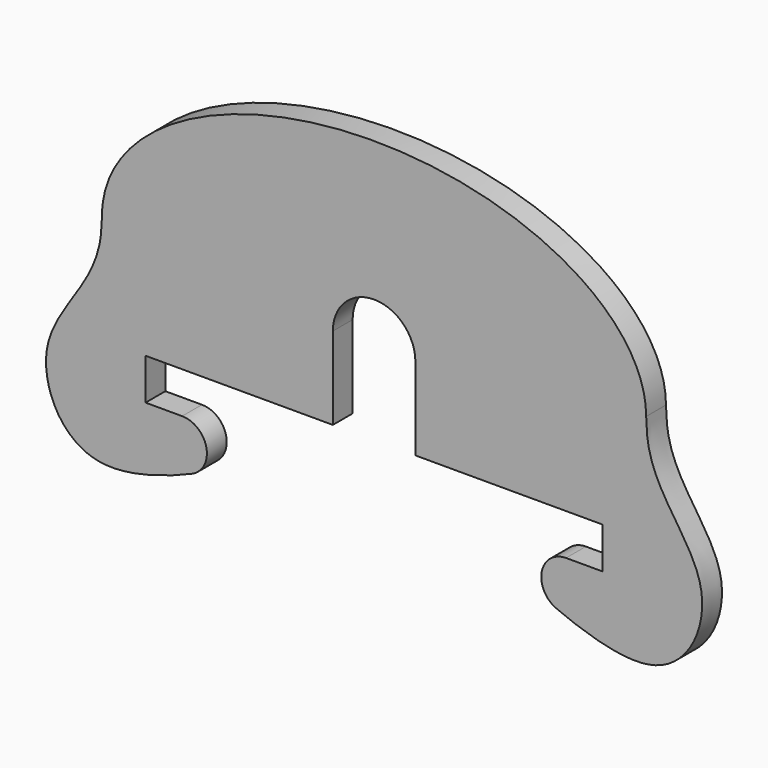
from build123d import *

# Parameters (mm, degrees)
F1_DEPTH = 3


# Not quite as in the source:
# - ends of sketch curves that miss each other by under 0.0002 mm in the source are joined
# - the dataset's text gives a spline's control points without its knots; the knots are read off the source's solid


with BuildPart() as f1:
    # F0 (on Front) → F1 (new body)
    with BuildSketch(Plane.XZ):
        with BuildLine():
            Line((-23.246137, -14.349078), (-27.68, -14.349078))
            Line((-27.68, -14.349078), (-27.68, -9.349078))
            Line((-27.68, -9.349078), (-5, -9.349078))
            Line((-5, -9.349078), (-5, 0.650922))
            ThreePointArc((-5, 0.650922), (0, 5.650922), (5, 0.650922))
            Line((5, 0.650922), (5, -9.349078))
            Line((5, -9.349078), (27.68, -9.349078))
            Line((27.68, -9.349078), (27.68, -14.349078))
            Line((27.68, -14.349078), (23.246138, -14.349078))
            ThreePointArc((23.246138, -14.349078), (20.3080963794, -16.7425209657), (22.0580781253, -20.1038037094))
            add(Edge.make_bspline(
                [(32.949969, 3.892538), (32.997769, 3.409313), (33.022006, -3.688842), (43.09044, -10.371035), (36.198633, -25.420185), (24.808451, -21.289985), (22.0580781253, -20.1038037094)],
                knots=[26.688985, 26.688985, 26.688985, 26.688985, 28.557776, 42.872008, 54.1154, 62.665306, 62.665306, 62.665306, 62.665306], degree=3))
            add(Edge.make_bspline(
                [(32.949969, 3.892538), (32.949969, 22.5609262335), (-5.7071e-06, 22.560923), (-32.9499804142, 22.5609197665), (-32.949969, 3.8925315331)],
                knots=[0, 0, 0, 1.5707965, 1.5707965, 3.141593, 3.141593, 3.141593], degree=2, weights=[1, 0.7071067199, 1, 0.7071067199, 1]))
            add(Edge.make_bspline(
                [(-32.949969, 3.8925315331), (-32.997769, 3.409313), (-33.022006, -3.688842), (-43.09044, -10.371035), (-36.198633, -25.420185), (-24.80845, -21.289985), (-22.058078, -20.103804)],
                knots=[26.688985, 26.688985, 26.688985, 26.688985, 28.557776, 42.872008, 54.1154, 62.665306, 62.665306, 62.665306, 62.665306], degree=3))
            ThreePointArc((-22.058078, -20.103804), (-20.3080952866, -16.7425214153), (-23.246137, -14.349078))
        make_face()
    extrude(amount=F1_DEPTH)


solid = f1.part
